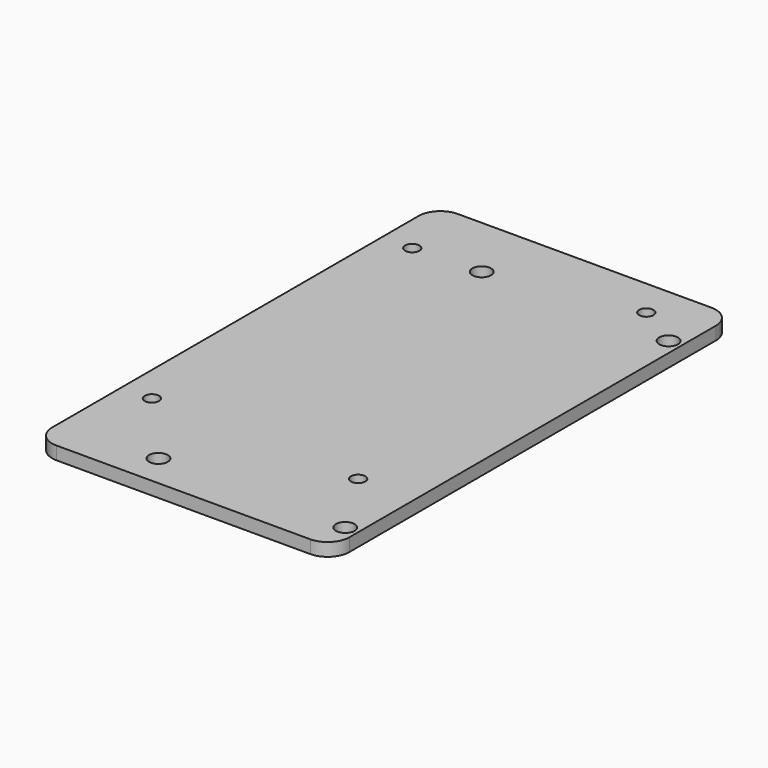
from build123d import *

# Parameters (mm, degrees)
F1_DEPTH = 3
F2_D     = 3.3
F3_D     = 4.3
F4_R     = 5


# Not quite as in the source:
# - a feature names something its author has since deleted; it is built from what else it names


with BuildPart() as f1:
    # F0 (on Top) → F1 (new body)
    with BuildSketch(Plane.XY):
        Polygon((-43.9476147294, -54.0188625455), (24.4538411498, -54.0188625455), (24.4538411498, 61.4031404257), (-43.9476147294, 61.4031404257), (-43.9476147294, 45.1967306435), align=None)
    extrude(amount=F1_DEPTH)

    # F2 (through all)
    with Locations(Plane(origin=(0, 0, 0), x_dir=(1, 0, 0), z_dir=(0, 0, -1))):
        with Locations((-37.0104938323, -45.9071589798), (11.4895061677, -52.6071589798), (11.4895061677, 30.2928410202), (-37.0104938323, 28.9928410202)):
            Hole(F2_D / 2)

    # F3 (through all)
    with Locations(Plane(origin=(0, 0, 0), x_dir=(1, 0, 0), z_dir=(0, 0, -1))):
        with Locations((-21.5, -46.5), (21.5, -46.5), (21.5, 46.5), (-21.5, 46.5)):
            Hole(F3_D / 2)

    # F4
    f4_edges = [f1.edges().sort_by_distance(p)[0] for p in [
        (-43.947615, -54.018863, 1.5),
        (24.453841, -54.018863, 1.5),
        (-43.947615, 61.40314, 1.5),
        (24.453841, 61.40314, 1.5),
    ]]
    fillet(f4_edges, radius=F4_R)


solid = f1.part
